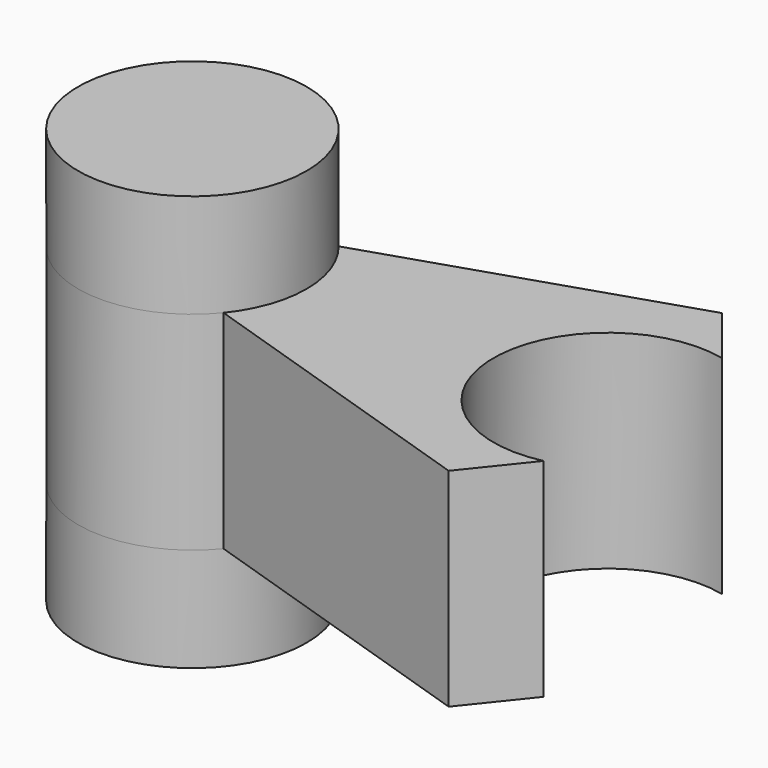
from build123d import *

# Parameters (mm, degrees)
F1_DEPTH = 2.5
F2_R     = 2.75
F3_DEPTH = 2.5


# Not quite as in the source:
# - a pattern or mirror of a feature is missing from the dataset's text; its kind, count and spacing are read off the source's solid


with BuildPart() as f1:
    # F0 (on Top) → F1 (new body, symmetric)
    with BuildSketch(Plane.XY):
        with BuildLine():
            Line((3.853342479, 2.6833219012), (2.7102889432, 4.112138821))
            Line((2.7102889432, 4.112138821), (-4.6141804357, 1.7322744554))
            ThreePointArc((-4.6141804357, 1.7322744554), (-9.5, 0), (-4.6141804357, -1.7322744554))
            Line((-4.6141804357, -1.7322744554), (2.7102889432, -4.112138821))
            Line((2.7102889432, -4.112138821), (3.853342479, -2.6833219012))
            Line((3.853342479, -2.6833219012), (3.853342479, -2.6829979227))
            ThreePointArc((3.853342479, -2.6829979227), (0.5, 0), (3.853342479, 2.6829979227))
            Line((3.853342479, 2.6829979227), (3.853342479, 2.6833219012))
        make_face()
    extrude(amount=F1_DEPTH, both=True)

    # F2 (on face) → F3 (join)
    with BuildSketch(Plane.XY.offset(2.5)):
        with Locations((-6.75, 0)):
            Circle(F2_R)
    f3 = extrude(amount=F3_DEPTH)

    # F3_copies: F3 across plane
    add(f3.mirror(Plane(origin=(0, 0, 0), x_dir=(-1, 0, 0), z_dir=(0, 0, -1))))


solid = f1.part
